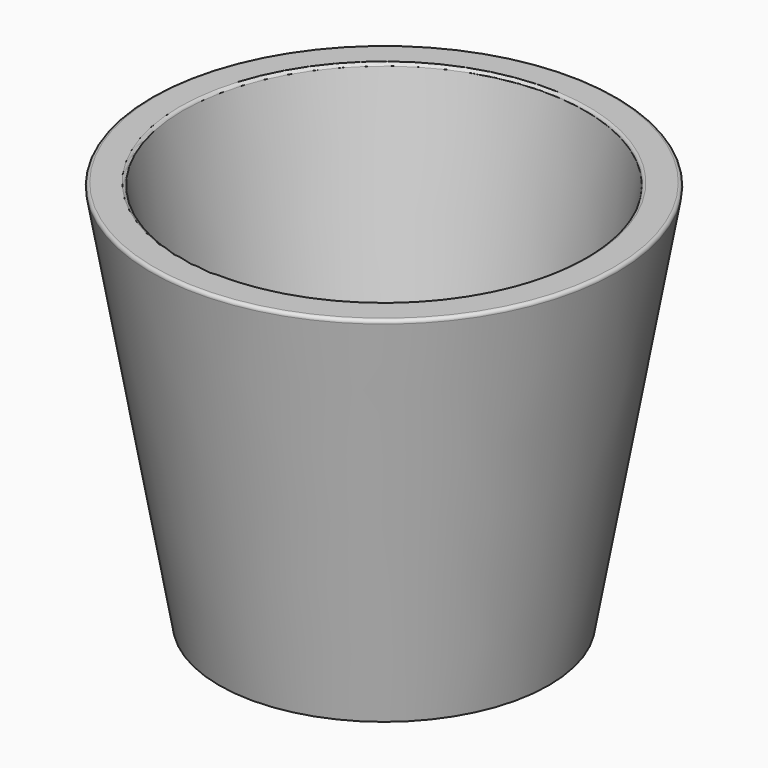
from build123d import *

# Parameters (mm, degrees)
F2_T = -5.08
F3_R = 0.508
F4_R = 0.508


# Not quite as in the source:
# - the program builds the solid bodies; features that only make, move or delete a surface that nothing else refers to are left out


with BuildPart() as f1:
    # F0 (on Front) → F1 (revolve)
    with BuildSketch(Plane.XZ):
        Polygon((0, 0), (0, 63.5), (-38.1, 63.5), (-26.903236725, 0), align=None)
    revolve(axis=Axis((0, 0, 31.75), (0, 0, 1)))

    # F2
    f2_openings = [f1.faces().sort_by_distance(p)[0] for p in [
        (0, 0, 63.5),
    ]]
    offset(amount=F2_T, openings=f2_openings)

    # F3
    f3_edges = [f1.edges().sort_by_distance(p)[0] for p in [
        (32.941633, 0, 63.5),
    ]]
    fillet(f3_edges, radius=F3_R)

    # F4
    f4_edges = [f1.edges().sort_by_distance(p)[0] for p in [
        (38.1, 0, 63.5),
    ]]
    fillet(f4_edges, radius=F4_R)


solid = f1.part
